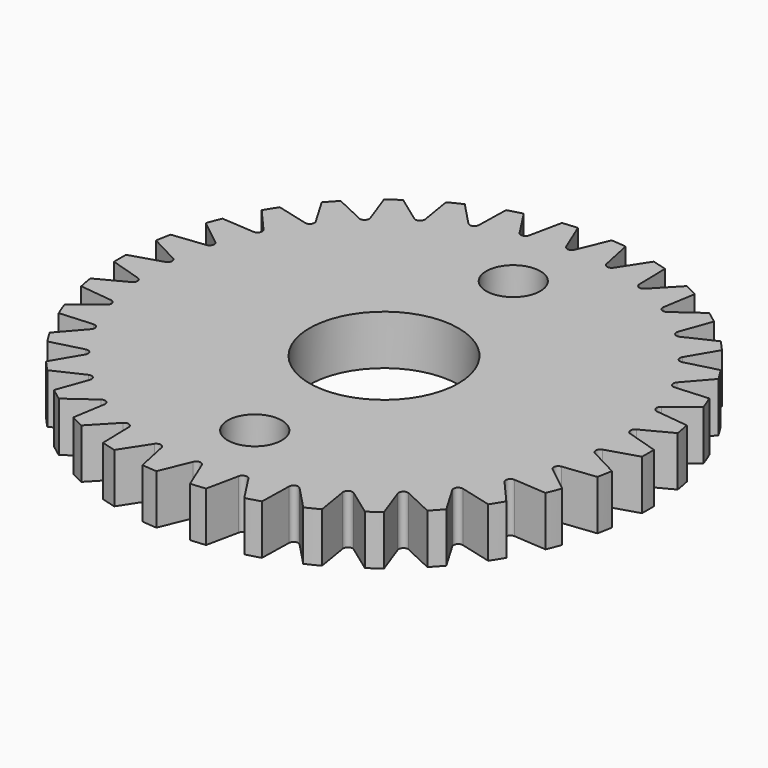
from build123d import *

# Parameters (mm, degrees)
F0_R            = 16.8606013276
F0_R_2          = 1.7272
F0_R_3          = 4.7625
F1_DEPTH        = 3.175
F3_DEPTH        = 3.175
F3_COPIES_COUNT = 34


# Not quite as in the source:
# - a pattern or mirror of a feature is missing from the dataset's text; its kind, count and spacing are read off the source's solid
# - a feature names something its author has since deleted; it is built from what else it names


with BuildPart() as f1:
    # F0 (on Top) → F1 (new body)
    with BuildSketch(Plane.XY):
        Circle(F0_R)
        with Locations((0, -10.31875)):
            Circle(F0_R_2, mode=Mode.SUBTRACT)
        Circle(F0_R_3, mode=Mode.SUBTRACT)
        with Locations((0, 10.31875)):
            Circle(F0_R_2, mode=Mode.SUBTRACT)
    extrude(amount=F1_DEPTH)

    # F2 (on face) → F3 (cut, through all)
    with BuildSketch(Plane.XY.offset(3.175)):
        with BuildLine():
            Line((0.2750051008, 14.882965874), (1.0776094804, 16.8261295293))
            ThreePointArc((1.0776094804, 16.8261295293), (0, 16.8606013276), (-1.0776094804, 16.8261295293))
            Line((-1.0776094804, 16.8261295293), (-0.2750051008, 14.882965874))
            ThreePointArc((-0.2750051008, 14.882965874), (0, 14.6990139664), (0.2750051008, 14.882965874))
        make_face()
    f3 = extrude(amount=-F3_DEPTH, mode=Mode.SUBTRACT)

    # F3_copies: F3 ×34 about axis
    f3_copies_axis = Axis((0, 0, 0), (0, 0, 1))
    for i in range(1, F3_COPIES_COUNT):
        add(f3.rotate(f3_copies_axis, i * 360 / F3_COPIES_COUNT), mode=Mode.SUBTRACT)


solid = f1.part
